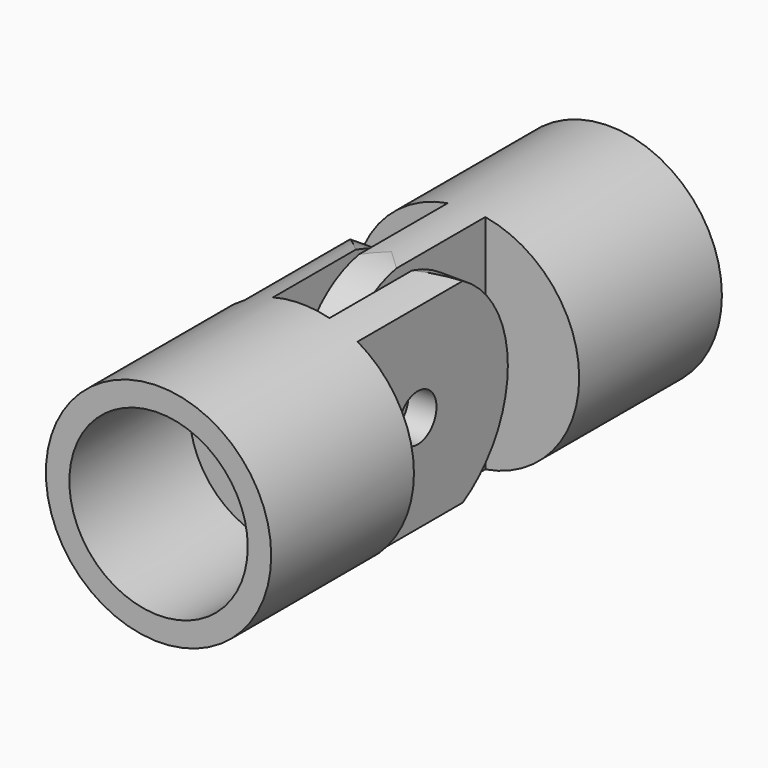
from build123d import *

# Parameters (mm, degrees)
F1_DEPTH  = 12
F3_R      = 5.99999
F4_R      = 5
F2_W      = 18.0606292561
F2_H      = 16.2687138654
F2_R      = 6
F5_DEPTH  = 35.7
F6_R      = 1.25
F7_DEPTH  = 25
F8_R      = 4.75
F9_DEPTH  = 8
F10_R     = 4.75
F11_DEPTH = 8


# Not quite as in the source:
# - a fillet or chamfer is up to 0.001 mm smaller than in the source, because OpenCascade refuses the exact size


with BuildPart() as f1:
    # F0 (on Top) → F1 (new body)
    with BuildSketch(Plane.XY):
        Polygon((6, 9.5), (-6, 9.5), (-6, 0), (-1, 0), (-1, -10), (1, -10), (1, 0), (6, 0), align=None)
    extrude(amount=F1_DEPTH)

    # F4
    f4_edges = [f1.edges().sort_by_distance(p)[0] for p in [
        (0, -10, 12),
        (0, -10, 0),
    ]]
    fillet(f4_edges, radius=F4_R)


with BuildPart() as f1b:
    # F0 (on Top) → F1, piece 2 (new body)
    with BuildSketch(Plane.XY):
        Polygon((-6, -11), (-6, -20.5), (6, -20.5), (6, -11), (3, -11), (3, -1), (1.5, -1), (1.5, -11), (-1.5, -11), (-1.5, -1), (-3, -1), (-3, -11), align=None)
    extrude(amount=F1_DEPTH)

    # F3 (radius 6 in the source; OpenCascade refuses exactly that, so slightly less here)
    f3_edges = [f1b.edges().sort_by_distance(p)[0] for p in [
        (2.25, -1, 12),
        (2.25, -1, 0),
        (-2.25, -1, 0),
        (-2.25, -1, 12),
    ]]
    fillet(f3_edges, radius=F3_R)


with BuildPart() as f5_tool:
    # F2 (on face) → F5 (new body)
    with BuildSketch(Plane.XZ.offset(20.5)):
        with Locations((0.2045785077, 5.5509812664)):
            Rectangle(F2_W, F2_H)
        with Locations((0, 6)):
            Circle(F2_R, mode=Mode.SUBTRACT)
    extrude(amount=-F5_DEPTH)


with BuildPart() as f1_1:
    add(f1.part)

    # F5: cut by f5_tool
    add(f5_tool.part, mode=Mode.SUBTRACT)


with BuildPart() as f1b_1:
    add(f1b.part)

    # F5: cut by f5_tool
    add(f5_tool.part, mode=Mode.SUBTRACT)


with BuildPart() as f7_tool:
    # F6 (on face) → F7 (new body)
    with BuildSketch(Plane.YZ.offset(3)):
        with Locations((-7, 6)):
            Circle(F6_R)
    extrude(amount=-F7_DEPTH)


with BuildPart() as f1_2:
    add(f1_1.part)

    # F7: cut by f7_tool
    add(f7_tool.part, mode=Mode.SUBTRACT)

    # F10 (on face) → F11 (cut)
    with BuildSketch(Plane(origin=(0, 9.5, 0), x_dir=(-1, 0, 0), z_dir=(0, 1, 0))):
        with Locations((0, 6)):
            Circle(F10_R)
    extrude(amount=-F11_DEPTH, mode=Mode.SUBTRACT)


with BuildPart() as f1b_2:
    add(f1b_1.part)

    # F7: cut by f7_tool
    add(f7_tool.part, mode=Mode.SUBTRACT)

    # F8 (on face) → F9 (cut)
    with BuildSketch(Plane.XZ.offset(20.5)):
        with Locations((0, 6)):
            Circle(F8_R)
    extrude(amount=-F9_DEPTH, mode=Mode.SUBTRACT)


solid = Compound([f1_2.part, f1b_2.part])
